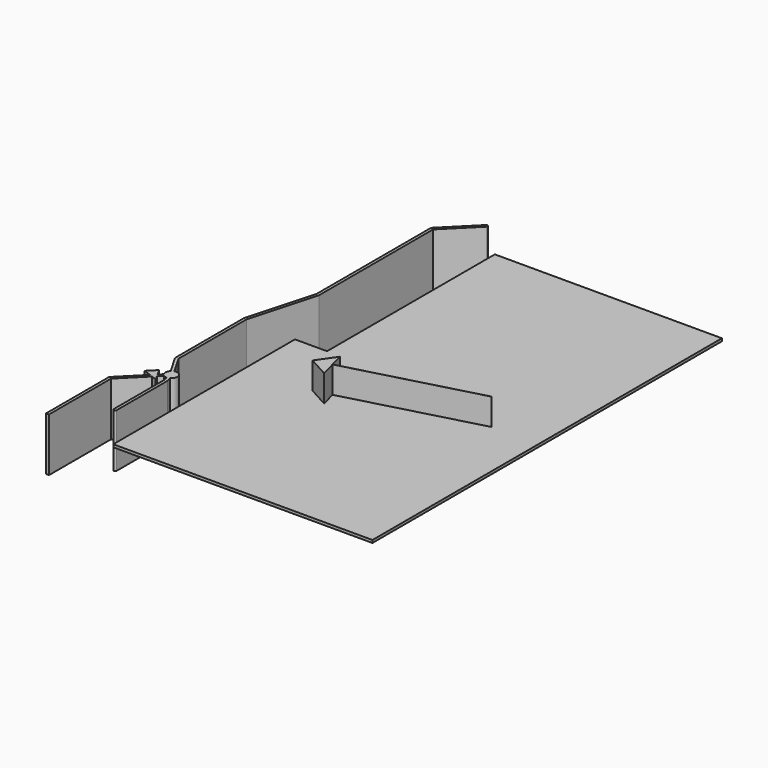
from build123d import *

# Parameters (mm, degrees)
F1_DEPTH      = 100
F3_DEPTH      = 1000
F3_DEPTH_BACK = 1000


# Not quite as in the source:
# - a feature names something its author has since deleted; it is built from what else it names


with BuildPart() as f1:
    # F0 (on Top) → F1 (new body)
    with BuildSketch(Plane.XY):
        Polygon((-843.9855575562, 913.8026237488), (-843.9855575561, -7586.1973762512), (8856.0144424439, -7586.1973762512), (8856.0144424438, 8763.8026237488), (356.0144424438, 8763.8026237488), (356.0144424438, 913.8026237488), align=None)
    extrude(amount=-F1_DEPTH)


with BuildPart() as f3:
    # F2 (on Top) → F3 (new body, two sides)
    with BuildSketch(Plane.XY) as f3_sk:
        with BuildLine():
            ThreePointArc((269.9053154091, 8474.9117507835), (281.827816732, 8492.7550349687), (286.0144424438, 8513.8026237488))
            ThreePointArc((286.0144424438, 8513.8026237488), (252.0620312239, 8564.6159980369), (192.1235694786, 8552.693496714))
            Line((192.1235694786, 8552.693496714), (269.9053154091, 8474.9117507835))
        make_face()
        with BuildLine():
            Line((269.9053154091, 8474.9117507835), (192.1235694786, 8552.693496714))
            ThreePointArc((192.1235694786, 8552.693496714), (192.1235694786, 8474.9117507835), (269.9053154091, 8474.9117507835))
        make_face()
        with BuildLine():
            ThreePointArc((269.9053154091, 8474.9117507835), (192.1235694786, 8474.9117507835), (192.1235694786, 8552.693496714))
            Line((192.1235694786, 8552.693496714), (-948.9855575562, 7411.5843696793))
            Line((-948.9855575562, 7411.5843696793), (-948.9855575562, 2043.63269294))
            Line((-948.9855575562, 2043.63269294), (-1648.9855575562, -480.6796410505))
            Line((-1648.9855575562, -480.6796410505), (-1648.9855575562, -3691.6079078613))
            Line((-1648.9855575562, -3691.6079078613), (-1225.7040759107, -4424.7529399743))
            ThreePointArc((-1225.7040759107, -4424.7529399743), (-1181.4855575561, -4391.3416603997), (-1130.4412814944, -4369.7529399743))
            Line((-1130.4412814944, -4369.7529399743), (-1538.9855575562, -3662.1334966938))
            Line((-1538.9855575562, -3662.1334966938), (-1538.9855575562, -495.6488760565))
            Line((-1538.9855575562, -495.6488760565), (-838.9855575562, 2028.663457934))
            Line((-838.9855575562, 2028.663457934), (-838.9855575562, 7366.0208778183))
            Line((-838.9855575562, 7366.0208778183), (269.9053154091, 8474.9117507835))
        make_face()
        with BuildLine():
            ThreePointArc((-1130.4412814944, -4369.7529399743), (-1181.4855575561, -4391.3416603997), (-1225.7040759107, -4424.7529399743))
            ThreePointArc((-1225.7040759107, -4424.7529399743), (-1292.0606513653, -4556.8289830017), (-1262.1489167268, -4701.5789894914))
            ThreePointArc((-1262.1489167268, -4701.5789894914), (-1228.0845833231, -4745.2964020182), (-1184.3671707963, -4779.3607354219))
            ThreePointArc((-1184.3671707963, -4779.3607354219), (-1127.2198427042, -4803.5306871663), (-1065.6438289459, -4811.1725589934))
            ThreePointArc((-1065.6438289459, -4811.1725589934), (-1010.7512724081, -4803.5306871663), (-959.3919880541, -4782.7024640322))
            ThreePointArc((-959.3919880541, -4782.7024640322), (-874.970670063, -4700.1413248883), (-843.9855575562, -4586.1973762512))
            ThreePointArc((-843.9855575562, -4586.1973762512), (-933.3436353604, -4406.6806111761), (-1130.4412814944, -4369.7529399743))
        make_face()
        with BuildLine():
            ThreePointArc((-1184.3671707963, -4779.3607354219), (-1228.0845833231, -4745.2964020182), (-1262.1489167268, -4701.5789894914))
            Line((-1262.1489167268, -4701.5789894914), (-1390.8192221094, -4830.249294874))
            Line((-1390.8192221094, -4830.249294874), (-1335.7238024601, -4930.7173670857))
            Line((-1335.7238024601, -4930.7173670857), (-1184.3671707963, -4779.3607354219))
        make_face()
        Polygon((-1335.7238024601, -4930.7173670857), (-1390.8192221094, -4830.249294874), (-1548.8158805226, -4988.2459532871), (-1435.3841341858, -5030.3776988114), align=None)
        Polygon((-1548.8158805226, -4988.2459532871), (-1390.8192221094, -4830.249294874), (-1527.3326635361, -4581.3131332397), (-1829.8729658127, -4883.8534355164), align=None)
        with BuildLine():
            Line((-913.9855575561, -4952.1615696408), (-959.3919880541, -4782.7024640322))
            ThreePointArc((-959.3919880541, -4782.7024640322), (-1010.7512724081, -4803.5306871663), (-1065.6438289459, -4811.1725589934))
            Line((-1065.6438289459, -4811.1725589934), (-1023.9855575561, -4966.6433443754))
            Line((-1023.9855575561, -4966.6433443754), (-1023.9855575561, -7336.1973762512))
            ThreePointArc((-1023.9855575561, -7336.1973762512), (-968.9855575561, -7281.1973762512), (-913.9855575561, -7336.1973762512))
            Line((-913.9855575561, -7336.1973762512), (-913.9855575561, -4952.1615696408))
        make_face()
        Polygon((-1241.6001558304, -5102.3545265198), (-1335.7238024601, -4930.7173670857), (-1435.3841341858, -5030.3776988114), align=None)
        Polygon((-1435.3841341858, -5030.3776988114), (-1548.8158805226, -4988.2459532871), (-2398.9855575561, -5838.4156303207), (-2398.9855575561, -8786.1973762512), (-2288.9855575561, -8786.1973762512), (-2288.9855575561, -5883.9791221817), align=None)
        with BuildLine():
            ThreePointArc((-1023.9855575561, -7336.1973762512), (-968.9855575561, -7391.1973762512), (-913.9855575561, -7336.1973762512))
            ThreePointArc((-913.9855575561, -7336.1973762512), (-968.9855575561, -7281.1973762512), (-1023.9855575561, -7336.1973762512))
        make_face()
    extrude(amount=-F3_DEPTH)
    extrude(f3_sk.sketch, amount=F3_DEPTH_BACK)


with BuildPart() as f3b:
    # F2 (on Top) → F3, piece 2 (new body, two sides)
    with BuildSketch(Plane.XY) as f3_2_sk:
        Polygon((7111.8739150801, 173.7785974403), (7111.3562769899, 175.7104490929), (2204.5480176534, -1139.0648614107), (2205.0656557436, -1140.9967130633), align=None)
        Polygon((2205.0656557436, -1140.9967130633), (2204.5480176534, -1139.0648614107), (1591.4141720975, -1303.3535801796), (1591.9318101877, -1305.2854318322), align=None)
        Polygon((1591.4141720975, -1303.3535801796), (2204.5480176534, -1139.0648614107), (2066.2712834871, -623.0090639974), align=None)
        Polygon((2362.4389377281, -1728.3217971832), (2205.0656557436, -1140.9967130633), (1591.9318101877, -1305.2854318322), align=None)
    extrude(amount=-F3_DEPTH)
    extrude(f3_2_sk.sketch, amount=F3_DEPTH_BACK)


solid = Compound([f1.part, f3.part, f3b.part])
